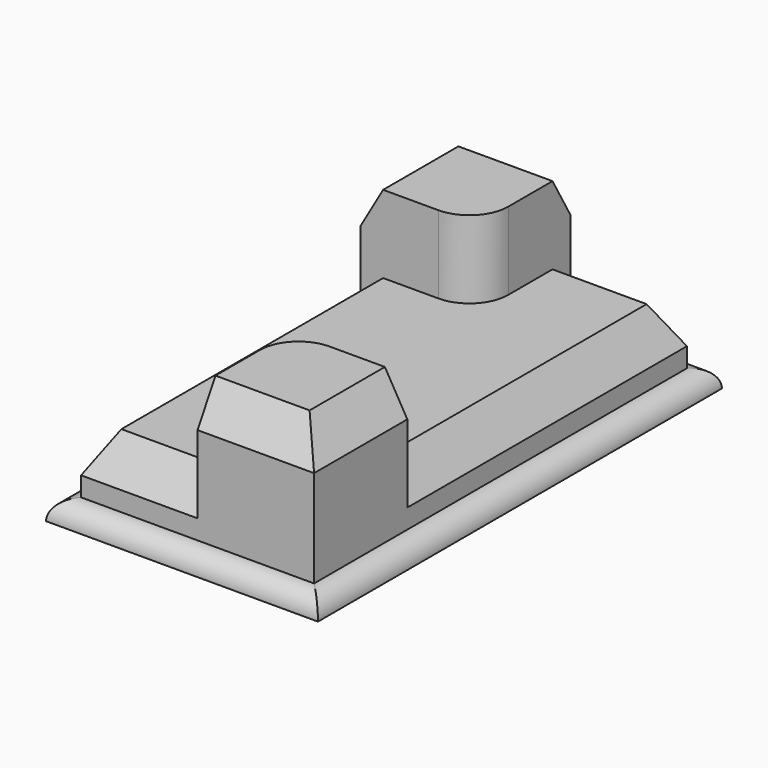
from build123d import *

# Parameters (mm, degrees)
F0_W     = 88.9
F0_H     = 165.1
F1_DEPTH = 6.35
F2_DEPTH = 25.4
F3_DEPTH = 50.8
F4_SIZE2 = 12.7
F4_SIZE  = 7.3323484187
F5_R     = 6.34999
F6_SIZE2 = 12.7
F6_SIZE  = 7.3323484187
F7_SIZE2 = 12.7
F7_SIZE  = 7.3323484187


# Not quite as in the source:
# - a fillet or chamfer is up to 0.001 mm smaller than in the source, because OpenCascade refuses the exact size


with BuildPart() as f1:
    # F0 (on Top) → F1 (new body)
    with BuildSketch(Plane.XY):
        Rectangle(F0_W, F0_H)
        Polygon((-38.1, 38.1), (-38.1, 76.2), (0, 76.2), (38.1, 76.2), (38.1, -38.1), (38.1, -76.2), (0, -76.2), (-38.1, -76.2), align=None, mode=Mode.SUBTRACT)
    extrude(amount=F1_DEPTH)

    # F0 (on Top) → F2 (join)
    with BuildSketch(Plane.XY):
        with BuildLine():
            Line((38.1, 76.2), (0, 76.2))
            Line((0, 76.2), (0, 50.8))
            ThreePointArc((0, 50.8), (-3.7197438789, 41.8197438789), (-12.7, 38.1))
            Line((-12.7, 38.1), (-38.1, 38.1))
            Line((-38.1, 38.1), (-38.1, -76.2))
            Line((-38.1, -76.2), (0, -76.2))
            Line((0, -76.2), (0, -50.8))
            ThreePointArc((0, -50.8), (3.7197438789, -41.8197438789), (12.7, -38.1))
            Line((12.7, -38.1), (38.1, -38.1))
            Line((38.1, -38.1), (38.1, 76.2))
        make_face()
    extrude(amount=F2_DEPTH)

    # F0 (on Top) → F3 (join)
    with BuildSketch(Plane.XY):
        with BuildLine():
            Line((38.1, -76.2), (38.1, -38.1))
            Line((38.1, -38.1), (12.7, -38.1))
            ThreePointArc((12.7, -38.1), (3.7197438789, -41.8197438789), (0, -50.8))
            Line((0, -50.8), (0, -76.2))
            Line((0, -76.2), (38.1, -76.2))
        make_face()
        with BuildLine():
            Line((0, 76.2), (-38.1, 76.2))
            Line((-38.1, 76.2), (-38.1, 38.1))
            Line((-38.1, 38.1), (-12.7, 38.1))
            ThreePointArc((-12.7, 38.1), (-3.7197438789, 41.8197438789), (0, 50.8))
            Line((0, 50.8), (0, 76.2))
        make_face()
    extrude(amount=F3_DEPTH)

    # F4
    f4_edges = [f1.edges().sort_by_distance(p)[0] for p in [
        (19.05, -76.2, 50.8),
        (38.1, -57.15, 50.8),
    ]]
    f4_side = f1.faces().sort_by_distance((19.446042, -57.546042, 50.8))[0]
    chamfer(f4_edges, length=F4_SIZE, length2=F4_SIZE2, reference=f4_side)

    # F5 (radius 6.35 in the source; OpenCascade refuses exactly that, so slightly less here)
    f5_edges = [f1.edges().sort_by_distance(p)[0] for p in [
        (0, -82.55, 6.35),
        (44.45, 0, 6.35),
        (0, 82.55, 6.35),
        (-44.45, 0, 6.35),
    ]]
    fillet(f5_edges, radius=F5_R)

    # F6
    f6_edges = [f1.edges().sort_by_distance(p)[0] for p in [
        (-19.05, 76.2, 50.8),
        (-38.1, 57.15, 50.8),
    ]]
    f6_side = f1.faces().sort_by_distance((-19.446042, 57.546042, 50.8))[0]
    chamfer(f6_edges, length=F6_SIZE, length2=F6_SIZE2, reference=f6_side)

    # F7
    f7_edges = [f1.edges().sort_by_distance(p)[0] for p in [
        (38.1, 19.05, 25.4),
        (19.05, 76.2, 25.4),
        (-38.1, -19.05, 25.4),
        (-19.05, -76.2, 25.4),
    ]]
    f7_side = f1.faces().sort_by_distance((0, 0, 25.4))[0]
    chamfer(f7_edges, length=F7_SIZE, length2=F7_SIZE2, reference=f7_side)


solid = f1.part
